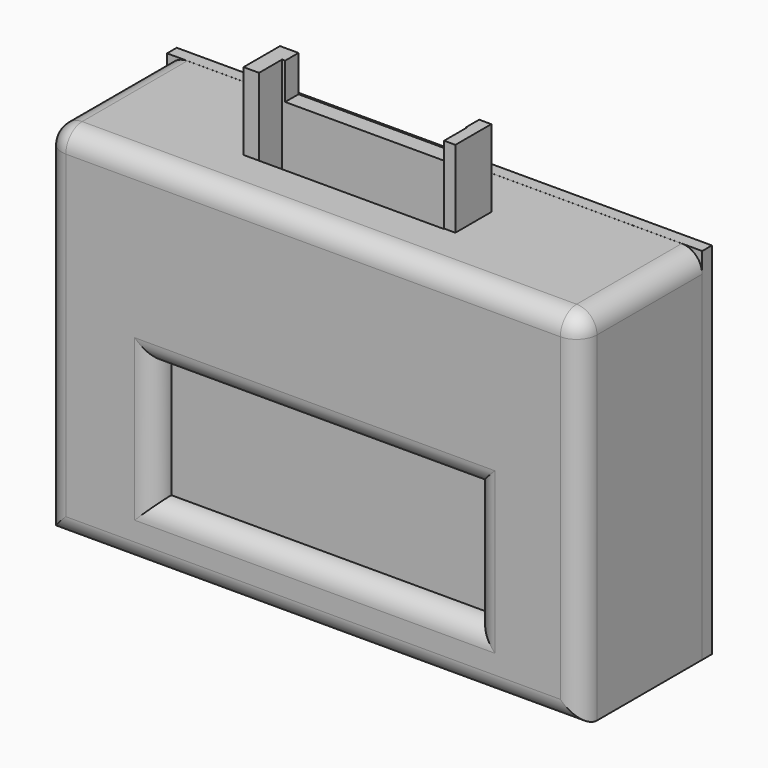
from build123d import *

# Parameters (mm, degrees)
F0_W          = 131.4388513565
F0_H          = 88.3812978864
F1_DEPTH      = 37.3
F2_W          = 78.4667283297
F2_H          = 29.4604320079
F3_DEPTH      = 61.4
F4_R          = 5
F5_W          = 131.4388513565
F5_H          = 88.3812978864
F6_DEPTH      = 3
F7_W          = 45.3237425536
F7_H          = 7.0818327367
F8_DEPTH      = 18.6
F9_W          = 39.392977953
F9_H          = 1.5654563904
F10_DEPTH     = 50.6
F11_T1_DEPTH  = 44.8
F11_S5_W      = 5
F11_S5_H      = 5
F11_T6_DEPTH  = 5
F11_S11_W     = 5
F11_S11_H     = 5
F11_T12_DEPTH = 5
F12_R         = 0.0241421356
F12_2_R       = 0.0241421356
F13_W         = 45.3237425536
F13_H         = 4.0992423892
F14_DEPTH     = 19
F15_W         = 3.8063414395
F15_H         = 11.1810751259
F16_DEPTH     = 19
F17_W         = 2.7666892856
F17_H         = 11.0205691308
F18_DEPTH     = 19
F19_W         = 44.3728975952
F19_H         = 8.9377077818
F20_DEPTH     = 25
F21_DEPTH     = 30.9


# Not quite as in the source:
# - a fillet or chamfer that OpenCascade refuses, or shapes differently, is made with other operations: its cross-section is extruded or revolved along the edge and cut away or added


with BuildPart() as f1:
    # F0 (on Front) → F1 (new body)
    with BuildSketch(Plane.XZ):
        Rectangle(F0_W, F0_H)
    extrude(amount=F1_DEPTH)

    # F2 (on face) → F3 (cut)
    with BuildSketch(Plane.XZ.offset(37.3)):
        with Locations((0.4249103367, -14.730216004)):
            Rectangle(F2_W, F2_H)
    extrude(amount=-F3_DEPTH, mode=Mode.SUBTRACT)

    # F4
    f4_edges = [f1.edges().sort_by_distance(p)[0] for p in [
        (0, -37.3, -44.190649),
        (-65.719426, -37.3, 0),
        (65.719426, -37.3, 0),
        (0, -37.3, 44.190649),
        (0.42491, -37.3, 0),
        (-38.808454, -37.3, -14.730216),
        (0.42491, -37.3, -29.460432),
        (39.658275, -37.3, -14.730216),
    ]]
    fillet(f4_edges, radius=F4_R)

    # F7 (on face) → F8 (cut)
    with BuildSketch(Plane.XY.offset(44.1906489432)):
        with Locations((-1.4163674787, -20.2540475875)):
            Rectangle(F7_W, F7_H)
    extrude(amount=-F8_DEPTH, mode=Mode.SUBTRACT)

    # F9 (on face) → F10 (cut)
    with BuildSketch(Plane.XY.offset(25.5906489432)):
        with Locations((-1.1046566069, -20.2819518745)):
            Rectangle(F9_W, F9_H)
    extrude(amount=-F10_DEPTH, mode=Mode.SUBTRACT)

    # F11: fillet of radius 5 on 2 edges, made by hand

    # F11_s2 → F11_t1 (cut)
    with BuildSketch(Plane.XZ.offset(-12.5)):
        with BuildLine():
            ThreePointArc((65.7194256783, 39.1906489432), (64.2549595842, 42.7261828491), (60.7194256783, 44.1906489432))
            Line((60.7194256783, 44.1906489432), (65.7194256783, 44.1906489432))
            Line((65.7194256783, 44.1906489432), (65.7194256783, 39.1906489432))
        make_face()
        with BuildLine():
            ThreePointArc((-65.7194256783, 39.1906489432), (-64.2549595842, 42.7261828491), (-60.7194256783, 44.1906489432))
            Line((-60.7194256783, 44.1906489432), (-65.7194256783, 44.1906489432))
            Line((-65.7194256783, 44.1906489432), (-65.7194256783, 39.1906489432))
        make_face()
    extrude(amount=F11_T1_DEPTH, mode=Mode.SUBTRACT)


with BuildPart() as f6:
    # F5 (on face) → F6 (new body)
    with BuildSketch(Plane(origin=(0, 0, 0), x_dir=(-1, 0, 0), z_dir=(0, 1, 0))):
        Rectangle(F5_W, F5_H)
    extrude(amount=F6_DEPTH)

    # F12
    f12_edges = [f6.edges().sort_by_distance(p)[0] for p in [
        (-65.719426, 3, 0),
        (0, 3, 44.190649),
        (65.719426, 3, 0),
        (0, 3, -44.190649),
    ]]
    fillet(f12_edges, radius=F12_R)


with BuildPart() as f11_tool4:
    # F11_s5 → F11_t6 (new body)
    with BuildSketch(Plane.YZ.offset(-60.7194256783)):
        with Locations((-34.8, 41.6906489432)):
            Rectangle(F11_S5_W, F11_S5_H)
    extrude(amount=-F11_T6_DEPTH)

    # F11_s7 → F11_t8 (revolve, cut)
    with BuildSketch(Plane(origin=(-60.7194256783, -32.3, 39.1906489432), x_dir=(0, 0.7071067812, -0.7071067812), z_dir=(0, 0.7071067812, 0.7071067812))):
        with BuildLine():
            ThreePointArc((0, -5), (5, 0), (0, 5))
            Line((0, 5), (0, -5))
        make_face()
    revolve(axis=Axis((-60.7194256783, -32.3, 39.1906489432), (-1, 0, 0)), mode=Mode.SUBTRACT)


with BuildPart() as f1_1:
    add(f1.part)

    # F11_t3: cut F11_tool4
    add(f11_tool4.part, mode=Mode.SUBTRACT)


with BuildPart() as f11_tool10:
    # F11_s11 → F11_t12 (new body)
    with BuildSketch(Plane.YZ.offset(60.7194256783)):
        with Locations((-34.8, 41.6906489432)):
            Rectangle(F11_S11_W, F11_S11_H)
    extrude(amount=F11_T12_DEPTH)

    # F11_s13 → F11_t14 (revolve, cut)
    with BuildSketch(Plane(origin=(60.7194256783, -32.3, 39.1906489432), x_dir=(0, 0.7071067812, -0.7071067812), z_dir=(0, -0.7071067812, -0.7071067812))):
        with BuildLine():
            ThreePointArc((0, -5), (5, 0), (0, 5))
            Line((0, 5), (0, -5))
        make_face()
    revolve(axis=Axis((60.7194256783, -32.3, 39.1906489432), (1, 0, 0)), mode=Mode.SUBTRACT)


with BuildPart() as f1_2:
    add(f1_1.part)

    # F11_t9: cut F11_tool10
    add(f11_tool10.part, mode=Mode.SUBTRACT)

    # F12#2
    f12_2_edges = [f1_2.edges().sort_by_distance(p)[0] for p in [
        (64.25496, 0, 42.726183),
        (-64.25496, 0, 42.726183),
    ]]
    fillet(f12_2_edges, radius=F12_2_R)

    # F13 (on face) → F14 (join)
    with BuildSketch(Plane.XY.offset(44.1906489432)):
        with Locations((-1.4163674787, -14.6635100245)):
            Rectangle(F13_W, F13_H)
    extrude(amount=F14_DEPTH)

    # F15 (on face) → F16 (join)
    with BuildSketch(Plane.XY.offset(44.1906489432)):
        with Locations((-25.9814094752, -18.2044263929)):
            Rectangle(F15_W, F15_H)
    extrude(amount=F16_DEPTH)

    # F17 (on face) → F18 (join)
    with BuildSketch(Plane.XY.offset(44.1906489432)):
        with Locations((22.6288484409, -18.1241733953)):
            Rectangle(F17_W, F17_H)
    extrude(amount=F18_DEPTH)

    # F19 (on face) → F20 (cut)
    with BuildSketch(Plane(origin=(0, -12.6138888299, 0), x_dir=(-1, 0, 0), z_dir=(0, 1, 0))):
        with Locations((1.1502206326, 58.7217950523)):
            Rectangle(F19_W, F19_H)
    extrude(amount=-F20_DEPTH, mode=Mode.SUBTRACT)


with BuildPart() as f21:
    # F21 (new): a face of the model
    f21_faces = [f1_2.part.faces().sort_by_distance(p)[0] for p in [
        (0.4249103367, -16.15, -29.4604320079),
    ]]
    extrude(f21_faces, amount=F21_DEPTH)


solid = Compound([f6.part, f1_2.part, f21.part])
